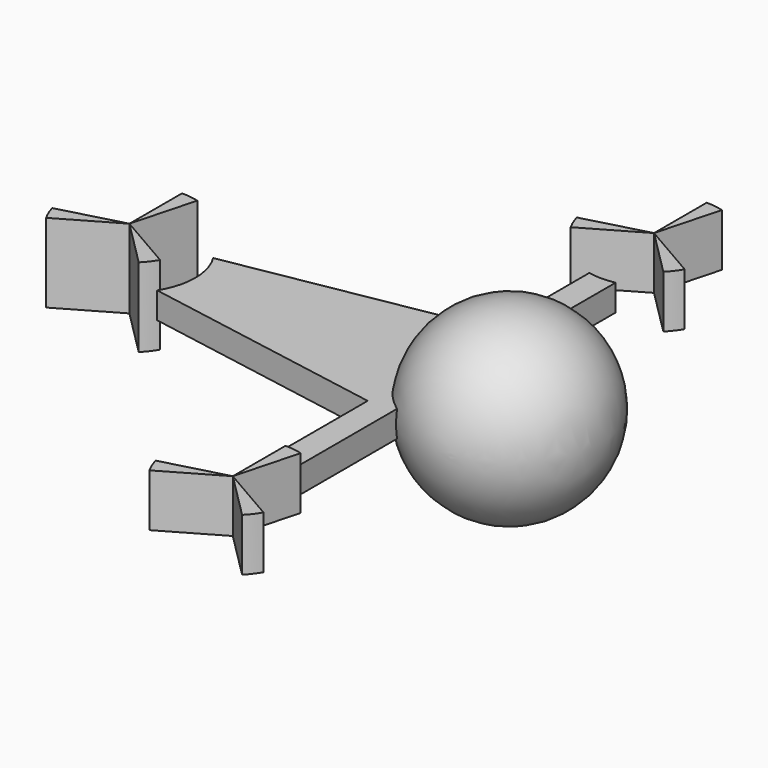
from build123d import *

# Parameters (mm, degrees)
F2_DEPTH  = 2.54
F3_DEPTH  = 5.08
F4_DEPTH  = 7.62
F8_DEPTH  = 25.4
F10_DEPTH = 22.861
F12_DEPTH = 25.401


# Not quite as in the source:
# - the program builds the solid bodies; features that only make, move or delete a surface that nothing else refers to are left out


with BuildPart() as f1:
    # F0 (on Top) → F1 (revolve)
    with BuildSketch(Plane.XY):
        with BuildLine():
            Line((0, 0), (0, -17.78))
            ThreePointArc((0, -17.78), (17.78, 0), (0, 17.78))
            Line((0, 17.78), (0, 0))
        make_face()
    revolve(axis=Axis((0, -8.89, 0), (0, -1, 0)))

    # F0 (on Top) → F2 (join, symmetric)
    with BuildSketch(Plane.XY):
        with BuildLine():
            Line((-15.24, 15.092776814), (-10.16, 15.988517876))
            Line((-10.16, 15.988517876), (-10.16, 38.3565921067))
            ThreePointArc((-10.16, 38.3565921067), (-12.7, 38.1), (-15.24, 38.3565921067))
            Line((-15.24, 38.3565921067), (-15.24, 15.092776814))
        make_face()
        Polygon((-15.24, -15.092776814), (-10.16, -15.988517876), (-10.16, 0), (-10.16, 15.988517876), (-15.24, 15.092776814), (-15.24, 0), align=None)
        with BuildLine():
            Line((-62.5352923163, -6.7533407181), (-15.24, -15.092776814))
            Line((-15.24, -15.092776814), (-15.24, 0))
            Line((-15.24, 0), (-15.24, 15.092776814))
            Line((-15.24, 15.092776814), (-62.5352923163, 6.7533407181))
            ThreePointArc((-62.5352923163, 6.7533407181), (-61.086650628, 3.5138440574), (-60.5908671101, 0))
            ThreePointArc((-60.5908671101, 0), (-61.086650628, -3.5138440574), (-62.5352923163, -6.7533407181))
        make_face()
        with BuildLine():
            Line((-10.16, -38.3565921067), (-10.16, -15.988517876))
            Line((-10.16, -15.988517876), (-15.24, -15.092776814))
            Line((-15.24, -15.092776814), (-15.24, -38.3565921067))
            ThreePointArc((-15.24, -38.3565921067), (-13.9764638175, -38.1643108568), (-12.7, -38.1))
            ThreePointArc((-12.7, -38.1), (-11.4235361825, -38.1643108568), (-10.16, -38.3565921067))
        make_face()
    extrude(amount=F2_DEPTH, both=True)


with BuildPart() as f3:
    # F0 (on Top) → F3 (new body, symmetric)
    with BuildSketch(Plane.XY):
        with BuildLine():
            Line((-10.16, 47.2073256969), (-10.16, 38.3565921067))
            ThreePointArc((-10.16, 38.3565921067), (-2.8626223006, 42.7678147432), (0, 50.8))
            ThreePointArc((0, 50.8), (-20.7321852568, 60.6373776994), (-15.24, 38.3565921067))
            Line((-15.24, 38.3565921067), (-15.24, 46.6368459165))
            Line((-15.24, 46.6368459165), (-10.16, 47.2073256969))
        make_face()
        with BuildLine():
            ThreePointArc((-15.24, 38.3565921067), (-12.7, 38.1), (-10.16, 38.3565921067))
            Line((-10.16, 38.3565921067), (-10.16, 47.2073256969))
            Line((-10.16, 47.2073256969), (-15.24, 46.6368459165))
            Line((-15.24, 46.6368459165), (-15.24, 38.3565921067))
        make_face()
    extrude(amount=F3_DEPTH, both=True)

    # F7 (on face) → F8 (cut)
    with BuildSketch(Plane.XY.offset(5.08)):
        with BuildLine():
            Line((-9.4129981272, 63.0672579939), (-12.7, 50.8))
            Line((-12.7, 50.8), (-1.7014773719, 44.45))
            ThreePointArc((-1.7014773719, 44.45), (-0.4327420061, 47.5129981272), (0, 50.8))
            ThreePointArc((0, 50.8), (-2.6244125783, 58.5312701484), (-9.4129981272, 63.0672579939))
        make_face()
        with BuildLine():
            Line((-24.9672579939, 47.5129981272), (-12.7, 50.8))
            Line((-12.7, 50.8), (-12.7, 63.5))
            ThreePointArc((-12.7, 63.5), (-22.7755874217, 58.5312701484), (-24.9672579939, 47.5129981272))
        make_face()
        with BuildLine():
            Line((-3.7197438789, 41.8197438789), (-12.7, 50.8))
            Line((-12.7, 50.8), (-23.6985226281, 44.45))
            ThreePointArc((-23.6985226281, 44.45), (-14.3576826412, 38.2086502606), (-3.7197438789, 41.8197438789))
        make_face()
    extrude(amount=-F8_DEPTH, mode=Mode.SUBTRACT)


with BuildPart() as f3b:
    # F0 (on Top) → F3, piece 2 (new body, symmetric)
    with BuildSketch(Plane.XY):
        with BuildLine():
            ThreePointArc((0, -50.8), (-2.8626223006, -42.7678147432), (-10.16, -38.3565921067))
            Line((-10.16, -38.3565921067), (-10.16, -45.2106446028))
            Line((-10.16, -45.2106446028), (-12.7, -44.8303223014))
            Line((-12.7, -44.8303223014), (-15.24, -44.45))
            Line((-15.24, -44.45), (-15.24, -38.3565921067))
            ThreePointArc((-15.24, -38.3565921067), (-20.7321852568, -60.6373776994), (0, -50.8))
        make_face()
        with BuildLine():
            ThreePointArc((-12.7, -38.1), (-13.9764638175, -38.1643108568), (-15.24, -38.3565921067))
            Line((-15.24, -38.3565921067), (-15.24, -44.45))
            Line((-15.24, -44.45), (-12.7, -44.8303223014))
            Line((-12.7, -44.8303223014), (-12.7, -38.1))
        make_face()
        with BuildLine():
            Line((-10.16, -45.2106446028), (-10.16, -38.3565921067))
            ThreePointArc((-10.16, -38.3565921067), (-11.4235361825, -38.1643108568), (-12.7, -38.1))
            Line((-12.7, -38.1), (-12.7, -44.8303223014))
            Line((-12.7, -44.8303223014), (-10.16, -45.2106446028))
        make_face()
    extrude(amount=F3_DEPTH, both=True)

    # F6 (on face) → F10 (cut, through all)
    with BuildSketch(Plane.XY.offset(5.08)):
        with BuildLine():
            Line((-9.4129981272, -38.5327420061), (-12.7, -50.8))
            Line((-12.7, -50.8), (-1.7014773719, -57.15))
            ThreePointArc((-1.7014773719, -57.15), (-0.4327420061, -54.0870018728), (0, -50.8))
            ThreePointArc((0, -50.8), (-2.6244125783, -43.0687298516), (-9.4129981272, -38.5327420061))
        make_face()
        with BuildLine():
            Line((-24.9672579939, -54.0870018728), (-12.7, -50.8))
            Line((-12.7, -50.8), (-12.7, -38.1))
            ThreePointArc((-12.7, -38.1), (-22.7755874217, -43.0687298516), (-24.9672579939, -54.0870018728))
        make_face()
        with BuildLine():
            Line((-3.7197438789, -59.7802561211), (-12.7, -50.8))
            Line((-12.7, -50.8), (-23.6985226281, -57.15))
            ThreePointArc((-23.6985226281, -57.15), (-14.3576826412, -63.3913497394), (-3.7197438789, -59.7802561211))
        make_face()
    extrude(amount=-F10_DEPTH, mode=Mode.SUBTRACT)


with BuildPart() as f4:
    # F0 (on Top) → F4 (new body, symmetric)
    with BuildSketch(Plane.XY):
        with BuildLine():
            ThreePointArc((-62.5352923163, 6.7533407181), (-85.9908671101, 0), (-62.5352923163, -6.7533407181))
            ThreePointArc((-62.5352923163, -6.7533407181), (-61.086650628, -3.5138440574), (-60.5908671101, 0))
            ThreePointArc((-60.5908671101, 0), (-61.086650628, 3.5138440574), (-62.5352923163, 6.7533407181))
        make_face()
    extrude(amount=F4_DEPTH, both=True)

    # F5 (on face) → F12 (cut, through all)
    with BuildSketch(Plane.XY.offset(7.62)):
        with BuildLine():
            Line((-85.5581251039, -3.2870018728), (-73.2908671101, 0))
            Line((-73.2908671101, 0), (-73.2908671101, 12.7))
            ThreePointArc((-73.2908671101, 12.7), (-83.3664545318, 7.7312701484), (-85.5581251039, -3.2870018728))
        make_face()
        with BuildLine():
            Line((-70.0038652373, 12.2672579939), (-73.2908671101, 0))
            Line((-73.2908671101, 0), (-62.292344482, -6.35))
            ThreePointArc((-62.292344482, -6.35), (-61.0236091162, -3.2870018728), (-60.5908671101, 0))
            ThreePointArc((-60.5908671101, 0), (-61.086650628, 3.5138440574), (-62.5352923163, 6.7533407181))
            ThreePointArc((-62.5352923163, 6.7533407181), (-65.7477039281, 10.2171761857), (-70.0038652373, 12.2672579939))
        make_face()
        with BuildLine():
            Line((-64.310610989, -8.9802561211), (-73.2908671101, 0))
            Line((-73.2908671101, 0), (-84.2893897381, -6.35))
            ThreePointArc((-84.2893897381, -6.35), (-74.9485497512, -12.5913497394), (-64.310610989, -8.9802561211))
        make_face()
    extrude(amount=-F12_DEPTH, mode=Mode.SUBTRACT)


solid = Compound([f1.part, f3.part, f3b.part, f4.part])
